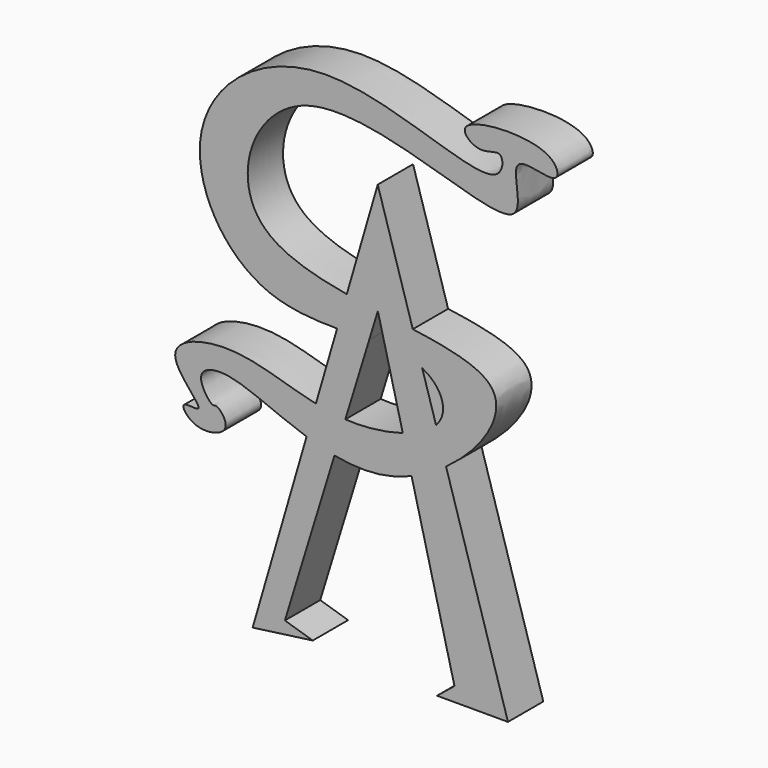
from build123d import *

# Parameters (mm, degrees)
F1_DEPTH = 10
F2_R     = 2.5
F3_DEPTH = 10


with BuildPart() as f1:
    # F0 (on Front) → F1 (new body)
    with BuildSketch(Plane.XZ):
        with BuildLine():
            add(Edge.make_bspline(
                [(-31.3811045376, 0.9740757505), (-38.2075651147, 2.4919536939), (-50.0914813356, 7.6780035275), (-69.2333093541, 2.0168539484), (-54.2945895273, -10.2829910385), (-63.0907202228, -7.7106938537), (-58.8127710183, -13.8461768887), (-49.4200741175, -11.4493464675), (-53.8533735403, -6.2281438394), (-54.8401337791, -7.5928356079), (-59.6268427844, -0.9997243163), (-54.5682626109, 0.6377264074), (-50.955273211, 0)],
                knots=[0.7680049296, 0.7680049296, 0.7680049296, 0.7680049296, 0.8043680213, 0.8381881962, 0.8675357674, 0.8841273645, 0.9029480805, 0.927287507, 0.9458949927, 0.9545418564, 0.9759316093, 1, 1, 1, 1], degree=3))
            add(Edge.make_bspline(
                [(-50.955273211, 0), (-46.3911044079, -0.8056184647), (-40.3353655324, -4.0124938693), (-33.4904909154, -6.2891722224)],
                knots=[0, 0, 0, 0, 0.0304047939, 0.0304047939, 0.0304047939, 0.0304047939], degree=3))
            add(Edge.make_bspline(
                [(-33.4904909154, -6.2891722224), (-31.4487320877, -6.9682830003), (-29.3367583079, -7.5646276101), (-27.1732128665, -7.9897860228)],
                knots=[0.0304047939, 0.0304047939, 0.0304047939, 0.0304047939, 0.0394742451, 0.0394742451, 0.0394742451, 0.0394742451], degree=3))
            add(Edge.make_bspline(
                [(-27.1732128665, -7.9897860228), (-23.1682300946, -8.7768053686), (-17.3291748235, -9.0566655751), (-11.3761352256, -7.0992742047), (-9.7135112686, -6.4006888907)],
                knots=[0.0394742451, 0.0394742451, 0.0394742451, 0.0394742451, 0.0562628899, 0.0629168188, 0.0629168188, 0.0629168188, 0.0629168188], degree=3))
            add(Edge.make_bspline(
                [(-9.7135112686, -6.4006888907), (-6.9827255519, -5.2532936608), (-4.3250031514, -3.7201323233), (-1.9010358024, -1.9662233489)],
                knots=[0.0629168188, 0.0629168188, 0.0629168188, 0.0629168188, 0.0738456004, 0.0738456004, 0.0738456004, 0.0738456004], degree=3))
            add(Edge.make_bspline(
                [(-1.9010358024, -1.9662233489), (6.1621044636, 3.8680194598), (15.8133854945, 18.4540345674), (-0.9363862321, 21.762799367), (-9.4359737664, 22.9512949984)],
                knots=[0.0738456004, 0.0738456004, 0.0738456004, 0.0738456004, 0.1101993487, 0.1379107077, 0.1379107077, 0.1379107077, 0.1379107077], degree=3))
            add(Edge.make_bspline(
                [(-9.4359737664, 22.9512949984), (-11.9916826173, 23.3086592578), (-14.66081128, 23.6440795333), (-17.3431764095, 24.008318521)],
                knots=[0.1379107077, 0.1379107077, 0.1379107077, 0.1379107077, 0.1462431316, 0.1462431316, 0.1462431316, 0.1462431316], degree=3))
            Line((-17.3431764095, 24.008318521), (-15.7209526392, 17.5427379558))
            add(Edge.make_bspline(
                [(-15.7209526392, 17.5427379558), (-12.7844443463, 17.427469513), (-9.8334805019, 17.0451250649), (-7.5320588401, 15.988819506), (-7.2943666736, 15.8691485651)],
                knots=[0.6682392351, 0.6682392351, 0.6682392351, 0.6682392351, 0.6827538761, 0.684486132, 0.684486132, 0.684486132, 0.684486132], degree=3))
            add(Edge.make_bspline(
                [(-7.2943666736, 15.8691485651), (-3.4589255263, 13.9381179473), (-1.2875634974, 9.4793065714), (-3.707293303, 6.068810456), (-4.1789132618, 5.5665597553)],
                knots=[0.684486132, 0.684486132, 0.684486132, 0.684486132, 0.7124381072, 0.7175814439, 0.7175814439, 0.7175814439, 0.7175814439], degree=3))
            add(Edge.make_bspline(
                [(-4.1789132618, 5.5665597553), (-5.7816094494, 3.8597717618), (-8.4879786378, 2.4737251762), (-11.6969991208, 1.5047559334)],
                knots=[0.7175814439, 0.7175814439, 0.7175814439, 0.7175814439, 0.7350599367, 0.7350599367, 0.7350599367, 0.7350599367], degree=3))
            add(Edge.make_bspline(
                [(-11.6969991208, 1.5047559334), (-15.6360404465, 0.3153556441), (-20.3480642345, -0.2474867064), (-24.7034993645, 0.0016429285), (-24.7179347993, 0.0024777518)],
                knots=[0.7350599367, 0.7350599367, 0.7350599367, 0.7350599367, 0.756514616, 0.7565859802, 0.7565859802, 0.7565859802, 0.7565859802], degree=3))
            add(Edge.make_bspline(
                [(-24.7179347993, 0.0024777518), (-27.0277425788, 0.1360574614), (-29.2374197136, 0.4974228973), (-31.3811045376, 0.9740757505)],
                knots=[0.7565859802, 0.7565859802, 0.7565859802, 0.7565859802, 0.7680049296, 0.7680049296, 0.7680049296, 0.7680049296], degree=3))
        make_face()
        with BuildLine():
            add(Edge.make_bspline(
                [(-33.4904909154, -6.2891722224), (-31.4487320877, -6.9682830003), (-29.3367583079, -7.5646276101), (-27.1732128665, -7.9897860228)],
                knots=[0.0304047939, 0.0304047939, 0.0304047939, 0.0304047939, 0.0394742451, 0.0394742451, 0.0394742451, 0.0394742451], degree=3))
            Line((-33.4904909154, -6.2891722224), (-45.6991418487, -48.3272075838))
            Line((-45.6991418487, -48.3272075838), (-32.0788043523, -46.4727090299))
            Line((-32.0788043523, -46.4727090299), (-38.3989587418, -44.5311143964))
            Line((-38.3989587418, -44.5311143964), (-27.1732128665, -7.9897860228))
        make_face()
        with BuildLine():
            Line((-26.5769480995, 17.5162227353), (-31.3811045376, 0.9740757505))
            add(Edge.make_bspline(
                [(-24.7179347993, 0.0024777518), (-27.0277425788, 0.1360574614), (-29.2374197136, 0.4974228973), (-31.3811045376, 0.9740757505)],
                knots=[0.7565859802, 0.7565859802, 0.7565859802, 0.7565859802, 0.7680049296, 0.7680049296, 0.7680049296, 0.7680049296], degree=3))
            Line((-24.7179347993, 0.0024777518), (-19.3141078758, 17.5926687535))
            add(Edge.make_bspline(
                [(-26.5769480995, 17.5162227353), (-24.0973740523, 17.5137238704), (-21.6465806753, 17.5818202397), (-19.3141078758, 17.5926687535)],
                knots=[0.6517416474, 0.6517416474, 0.6517416474, 0.6517416474, 0.6625270092, 0.6625270092, 0.6625270092, 0.6625270092], degree=3))
        make_face()
        with BuildLine():
            add(Edge.make_bspline(
                [(-24.3829712519, 25.0707409868), (-32.1065308991, 26.4055130206), (-53.5843263634, 32.381931904), (-38.9261309916, 76.3442783449), (21.5525657963, 42.0769367255), (10.3864460169, 67.5016391087), (24.5258020758, 61.086361949), (22.4966649095, 70.7764897276), (-2.2711428421, 69.1945270812), (5.7994007929, 62.3228875765), (11.285933405, 65.9896647627), (10.7209313744, 53.5413850755), (-31.4773471029, 77.385517799), (-66.4055963658, 48.4671413431), (-49.3042645472, 18.5689165996), (-31.8415777382, 17.5215283233), (-26.5769480995, 17.5162227353)],
                knots=[0.153571302, 0.153571302, 0.153571302, 0.153571302, 0.178058406, 0.2278872608, 0.2914998244, 0.3206660206, 0.3470826407, 0.3663311206, 0.4062790435, 0.4259693438, 0.4459579051, 0.4648481093, 0.5229237619, 0.5776113706, 0.6288421757, 0.6517416474, 0.6517416474, 0.6517416474, 0.6517416474], degree=3))
            add(Edge.make_bspline(
                [(-26.5769480995, 17.5162227353), (-24.0973740523, 17.5137238704), (-21.6465806753, 17.5818202397), (-19.3141078758, 17.5926687535)],
                knots=[0.6517416474, 0.6517416474, 0.6517416474, 0.6517416474, 0.6625270092, 0.6625270092, 0.6625270092, 0.6625270092], degree=3))
            Line((-19.3141078758, 17.5926687535), (-17.3431764095, 24.008318521))
            add(Edge.make_bspline(
                [(-17.3431764095, 24.008318521), (-19.7022533506, 24.3286581301), (-22.0715684184, 24.6712884025), (-24.3829712519, 25.0707409868)],
                knots=[0.1462431316, 0.1462431316, 0.1462431316, 0.1462431316, 0.153571302, 0.153571302, 0.153571302, 0.153571302], degree=3))
        make_face()
        with BuildLine():
            add(Edge.make_bspline(
                [(-9.7135112686, -6.4006888907), (-6.9827255519, -5.2532936608), (-4.3250031514, -3.7201323233), (-1.9010358024, -1.9662233489)],
                knots=[0.0629168188, 0.0629168188, 0.0629168188, 0.0629168188, 0.0738456004, 0.0738456004, 0.0738456004, 0.0738456004], degree=3))
            Line((-9.7135112686, -6.4006888907), (0, -45.1151318848))
            Line((0, -45.1151318848), (-3.9421002167, -48.3272075742))
            Line((-3.9421002167, -48.3272075742), (12.1183033315, -48.3272075742))
            Line((12.1183033315, -48.3272075742), (-1.9010358024, -1.9662233489))
        make_face()
        with BuildLine():
            Line((-15.7209526392, 17.5427379558), (-11.6969991208, 1.5047559334))
            add(Edge.make_bspline(
                [(-4.1789132618, 5.5665597553), (-5.7816094494, 3.8597717618), (-8.4879786378, 2.4737251762), (-11.6969991208, 1.5047559334)],
                knots=[0.7175814439, 0.7175814439, 0.7175814439, 0.7175814439, 0.7350599367, 0.7350599367, 0.7350599367, 0.7350599367], degree=3))
            Line((-4.1789132618, 5.5665597553), (-7.2943666736, 15.8691485651))
            add(Edge.make_bspline(
                [(-15.7209526392, 17.5427379558), (-12.7844443463, 17.427469513), (-9.8334805019, 17.0451250649), (-7.5320588401, 15.988819506), (-7.2943666736, 15.8691485651)],
                knots=[0.6682392351, 0.6682392351, 0.6682392351, 0.6682392351, 0.6827538761, 0.684486132, 0.684486132, 0.684486132, 0.684486132], degree=3))
        make_face()
        with BuildLine():
            Line((-17.3744335002, 49.2032319105), (-24.3829712519, 25.0707409868))
            add(Edge.make_bspline(
                [(-17.3431764095, 24.008318521), (-19.7022533506, 24.3286581301), (-22.0715684184, 24.6712884025), (-24.3829712519, 25.0707409868)],
                knots=[0.1462431316, 0.1462431316, 0.1462431316, 0.1462431316, 0.153571302, 0.153571302, 0.153571302, 0.153571302], degree=3))
            add(Edge.make_bspline(
                [(-9.4359737664, 22.9512949984), (-11.9916826173, 23.3086592578), (-14.66081128, 23.6440795333), (-17.3431764095, 24.008318521)],
                knots=[0.1379107077, 0.1379107077, 0.1379107077, 0.1379107077, 0.1462431316, 0.1462431316, 0.1462431316, 0.1462431316], degree=3))
            Line((-9.4359737664, 22.9512949984), (-17.3744335002, 49.2032319105))
        make_face()
    extrude(amount=F1_DEPTH)

    # F2 (on face) → F3 (join)
    with BuildSketch(Plane.XZ.offset(10)):
        with Locations((-36.6211347282, 62.411505729)):
            Circle(F2_R)
    extrude(amount=-F3_DEPTH)


solid = f1.part
